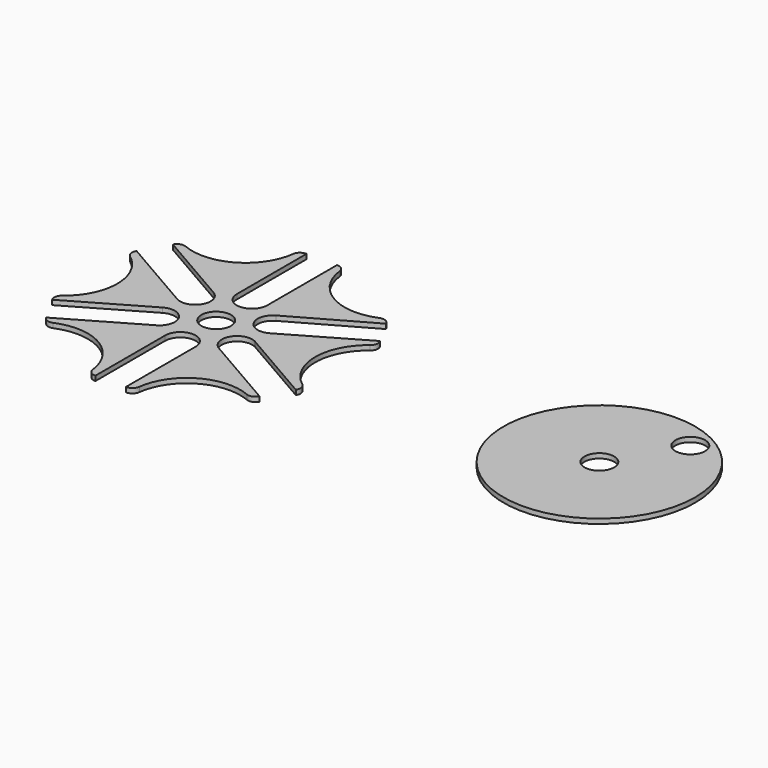
from build123d import *

# Parameters (mm, degrees)
F0_R     = 9.906
F1_DEPTH = 3.175
F2_R     = 5.08
F0_R_2   = 63.9582216699
F0_R_3   = 33.02
F3_DEPTH = 3.175


# Not quite as in the source:
# - a length typed as a fraction of an inch, garbled in the dataset ("3 / 203.2 mm" for 3/8 in), is restored
# - a feature names something its author has since deleted; it is built from what else it names


with BuildPart() as f1:
    # F0 (on Top) → F1 (new body)
    with BuildSketch(Plane.XY):
        with BuildLine():
            ThreePointArc((-17.78, -30.7958633586), (-35.5599563921, -0.0556901267), (-17.8763707949, 30.7400222382))
            Line((-17.8763707949, 30.7400222382), (-20.4296415334, 35.1306001794))
            Line((-20.4296415334, 35.1306001794), (-70.6329627114, 6.1469720917))
            ThreePointArc((-70.6329627114, 6.1469720917), (-84.5232381264, 9.8860746707), (-80.7525608015, 23.7678120156))
            ThreePointArc((-80.7525608015, 23.7678120156), (-80.7108842522, 23.7914906594), (-80.6690964546, 23.8149724163))
            Line((-80.6690964546, 23.8149724163), (-30.2104125797, 52.3259695061))
            Line((-30.2104125797, 52.3259695061), (-33.0188105519, 57.1902574851))
            ThreePointArc((-33.0188105519, 57.1902574851), (-68.5788105527, 57.1902574837), (-86.3588105535, 87.9861208428))
            Line((-86.3588105535, 87.9861208428), (-91.4394053355, 87.9861208428))
            Line((-91.4394053355, 87.9861208428), (-91.4394053355, 29.8429398183))
            ThreePointArc((-91.4394053355, 29.8429398183), (-101.6004354264, 19.6829398705), (-111.7594051266, 29.845))
            Line((-111.7594051266, 29.845), (-111.7594051266, 87.9881810245))
            Line((-111.7594051266, 87.9881810245), (-116.84, 87.9881810245))
            ThreePointArc((-116.84, 87.9881810245), (-134.62, 57.1923176659), (-170.18, 57.1923176659))
            Line((-170.18, 57.1923176659), (-172.7201599914, 52.7926315014))
            Line((-172.7201599914, 52.7926315014), (-122.4365198362, 23.7613583219))
            ThreePointArc((-122.4365198362, 23.7613583219), (-118.627620527, 9.8774561073), (-132.5265281759, 6.1236818976))
            Line((-132.5265281759, 6.1236818976), (-182.88, 35.1952724098))
            Line((-182.88, 35.1952724098), (-185.42, 30.7958633586))
            ThreePointArc((-185.42, 30.7958633586), (-167.64, 0), (-185.42, -30.7958633586))
            Line((-185.42, -30.7958633586), (-182.8800000009, -35.1952724082))
            Line((-182.8800000009, -35.1952724082), (-132.5258080212, -6.1245428478))
            ThreePointArc((-132.5258080212, -6.1245428478), (-118.6470606402, -9.8436248763), (-122.3661426686, -23.7223722573))
            Line((-122.3661426686, -23.7223722573), (-172.7194471607, -52.7938661604))
            Line((-172.7194471607, -52.7938661604), (-170.18, -57.1923176659))
            ThreePointArc((-170.18, -57.1923176659), (-134.62, -57.1923176659), (-116.84, -87.9881810245))
            Line((-116.84, -87.9881810245), (-111.76, -87.9881810245))
            Line((-111.76, -87.9881810245), (-111.76, -29.845))
            ThreePointArc((-111.76, -29.845), (-101.6, -19.685), (-91.44, -29.845))
            Line((-91.44, -29.845), (-91.4399999997, -87.9881810245))
            Line((-91.4399999997, -87.9881810245), (-86.36, -87.9881810245))
            ThreePointArc((-86.36, -87.9881810245), (-68.58, -57.1923176659), (-33.02, -57.1923176659))
            Line((-33.02, -57.1923176659), (-30.4777274407, -52.7889724266))
            Line((-30.4777274407, -52.7889724266), (-80.5680413022, -23.8693162349))
            ThreePointArc((-80.5680413022, -23.8693162349), (-84.7865541797, -10.2717986383), (-71.2681836795, -5.8061525812))
            ThreePointArc((-71.2681836795, -5.8061525812), (-70.6734718241, -6.1236818976), (-70.1011274419, -6.4799528141))
            Line((-70.1011274419, -6.4799528141), (-20.3311837367, -35.2146432099))
            Line((-20.3311837367, -35.2146432099), (-17.78, -30.7958633586))
        make_face()
        with Locations((-101.6, 0)):
            Circle(F0_R, mode=Mode.SUBTRACT)
    extrude(amount=F1_DEPTH)

    # F2
    f2_edges = [f1.edges().sort_by_distance(p)[0] for p in [
        (-17.876371, 30.740022, 1.5875),
        (-17.78, -30.795863, 1.5875),
        (-33.02, -57.192318, 1.5875),
        (-86.36, -87.988181, 1.5875),
        (-116.84, -87.988181, 1.5875),
        (-170.18, -57.192318, 1.5875),
        (-185.42, -30.795863, 1.5875),
        (-185.42, 30.795863, 1.5875),
        (-116.84, 87.988181, 1.5875),
        (-86.358811, 87.986121, 1.5875),
        (-33.018811, 57.190257, 1.5875),
        (-170.18, 57.192318, 1.5875),
    ]]
    fillet(f2_edges, radius=F2_R)


with BuildPart() as f3:
    # F0 (on Top) → F3 (new body)
    with BuildSketch(Plane.XY):
        with Locations((153.9702564478, 0)):
            Circle(F0_R_2)
        with Locations((153.9702564478, 0)):
            Circle(F0_R_3, mode=Mode.SUBTRACT)
        with Locations((179.5079290119, 43.9143174831)):
            Circle(F0_R, mode=Mode.SUBTRACT)
        with Locations((153.9702564478, 0)):
            Circle(F0_R_3)
        with Locations((153.9702564478, 0)):
            Circle(F0_R, mode=Mode.SUBTRACT)
    extrude(amount=F3_DEPTH)


solid = Compound([f1.part, f3.part])
